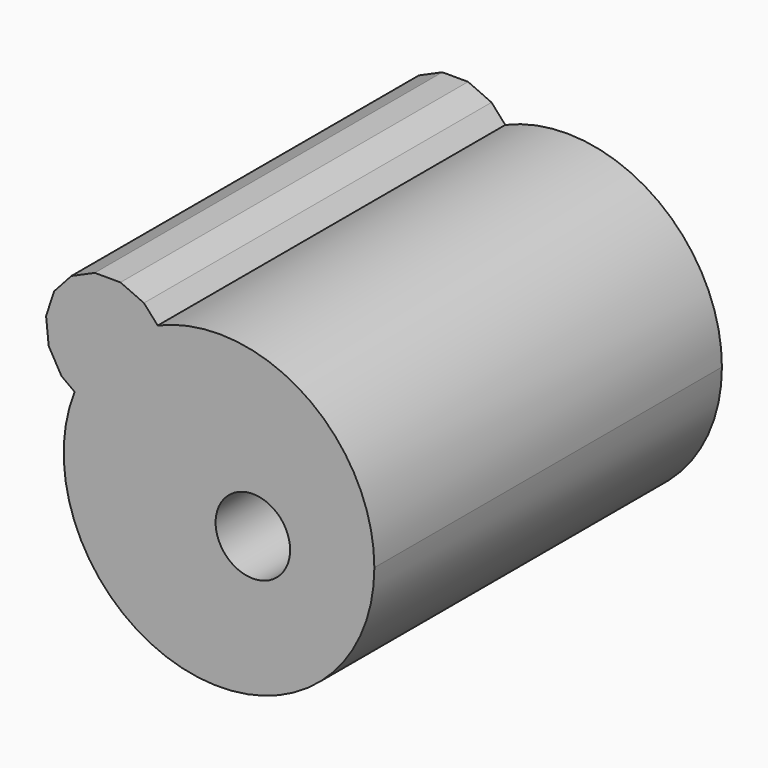
from build123d import *

# Parameters (mm, degrees)
F0_R     = 4.3560889736
F1_DEPTH = 50.8


with BuildPart() as f1:
    # F0 (on Front) → F1 (new body)
    with BuildSketch(Plane.XZ):
        with BuildLine():
            ThreePointArc((-50.8035481042, 44.8743139746), (-37.3327925125, 20.3368670349), (-15.7611440911, 38.1753519177))
            ThreePointArc((-15.7611440911, 38.1753519177), (-23.931762198, 53.3418471705), (-41.0919163358, 54.8619420575))
            Line((-41.0919163358, 54.8619420575), (-40.6960048204, 54.4206382187))
            Line((-40.6960048204, 54.4206382187), (-39.7726875247, 51.561406541))
            Line((-39.7726875247, 51.561406541), (-40.0921494975, 48.5738214521))
            Line((-40.0921494975, 48.5738214521), (-41.5991528616, 45.9744635553))
            Line((-41.5991528616, 45.9744635553), (-44.0331230447, 44.2127854453))
            Line((-44.0331230447, 44.2127854453), (-46.97320449, 43.5933972717))
            Line((-46.97320449, 43.5933972717), (-49.9110304061, 44.2233968767))
            Line((-49.9110304061, 44.2233968767), (-50.8035481042, 44.8743139746))
        make_face()
        with Locations((-29.9666635692, 36.7907546461)):
            Circle(F0_R, mode=Mode.SUBTRACT)
        with BuildLine():
            Line((-40.6960048204, 54.4206382187), (-41.0919163358, 54.8619420575))
            ThreePointArc((-41.0919163358, 54.8619420575), (-46.9434332236, 50.8363139975), (-50.8035481042, 44.8743139746))
            Line((-50.8035481042, 44.8743139746), (-49.9110304061, 44.2233968767))
            Line((-49.9110304061, 44.2233968767), (-46.97320449, 43.5933972717))
            Line((-46.97320449, 43.5933972717), (-44.0331230447, 44.2127854453))
            Line((-44.0331230447, 44.2127854453), (-41.5991528616, 45.9744635553))
            Line((-41.5991528616, 45.9744635553), (-40.0921494975, 48.5738214521))
            Line((-40.0921494975, 48.5738214521), (-39.7726875247, 51.561406541))
            Line((-39.7726875247, 51.561406541), (-40.6960048204, 54.4206382187))
        make_face()
        with BuildLine():
            ThreePointArc((-50.8035481042, 44.8743139746), (-46.9434332236, 50.8363139975), (-41.0919163358, 54.8619420575))
            Line((-41.0919163358, 54.8619420575), (-42.7024514363, 56.6571293527))
            Line((-42.7024514363, 56.6571293527), (-45.4450945244, 57.8841703083))
            Line((-45.4450945244, 57.8841703083), (-48.4497061786, 57.8895945568))
            Line((-48.4497061786, 57.8895945568), (-51.1967617479, 56.6724641964))
            Line((-51.1967617479, 56.6724641964), (-53.2112703682, 54.4432321237))
            Line((-53.2112703682, 54.4432321237), (-54.1449051977, 51.587352816))
            Line((-54.1449051977, 51.587352816), (-53.8362322927, 48.5986337504))
            Line((-53.8362322927, 48.5986337504), (-52.3386240026, 45.9938516051))
            Line((-52.3386240026, 45.9938516051), (-50.8035481042, 44.8743139746))
        make_face()
    extrude(amount=F1_DEPTH)


solid = f1.part
